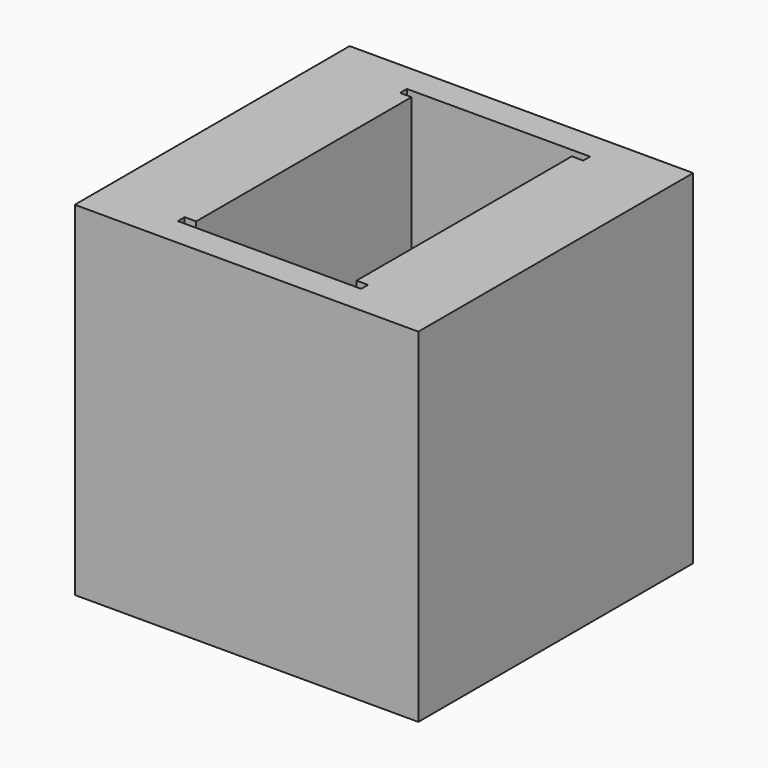
from build123d import *

# Parameters (mm, degrees)
F0_W     = 76.2
F0_H     = 76.2
F0_W_2   = 2.54
F0_H_2   = 59.69
F1_DEPTH = 76.2


# Not quite as in the source:
# - the program builds the solid bodies; features that only make, move or delete a surface that nothing else refers to are left out


with BuildPart() as f1:
    # F0 (on Top) → F1 (new body)
    with BuildSketch(Plane.XY):
        with Locations((-38.1, 38.1)):
            Rectangle(F0_W, F0_H)
        Polygon((-58.42, 69.85), (-17.78, 69.85), (-17.78, 67.945), (-17.78, 8.255), (-17.78, 6.35), (-58.42, 6.35), (-58.42, 8.255), (-58.42, 67.945), align=None, mode=Mode.SUBTRACT)
        with Locations((-57.15, 38.1)):
            Rectangle(F0_W_2, F0_H_2)
        with Locations((-19.05, 38.1)):
            Rectangle(F0_W_2, F0_H_2)
    extrude(amount=F1_DEPTH)


with BuildPart() as f1_1:
    # F3: moved
    add(f1.part.moved(Location((0, 106.934, 0))))


with BuildPart() as f1_2:
    # F6: moved
    add(f1_1.part.moved(Location((38.1, -144.526, 11.938))))


solid = f1_2.part
